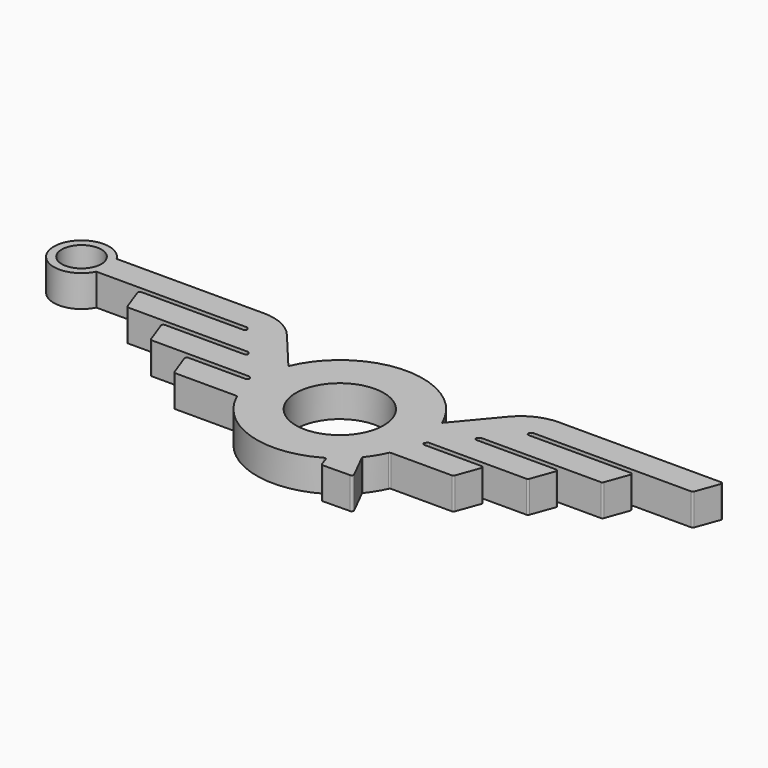
from build123d import *

# Parameters (mm, degrees)
F0_R     = 11.1
F1_DEPTH = 4
F2_DEPTH = 4
F3_DEPTH = 4
F4_DEPTH = 4
F5_R     = 0.5
F6_R     = 7
F6_R_2   = 5
F7_DEPTH = 4
F8_R     = 5
F9_DEPTH = 25
F10_R    = 12


# Not quite as in the source:
# - a feature names something its author has since deleted; it is built from what else it names


with BuildPart() as f1:
    # F0 (on Top) → F1 (new body, symmetric)
    with BuildSketch(Plane.XY):
        with BuildLine():
            ThreePointArc((20.944924, -1.519927), (20.986226, -0.760462), (21, 0))
            ThreePointArc((21, 0), (20.598026, 4.089169), (19.407495, 8.021792))
            ThreePointArc((19.407495, 8.021792), (0, 21), (-19.407495, 8.021792))
            ThreePointArc((-19.407495, 8.021792), (-20.732595, 3.340581), (-20.944924, -1.519927))
            ThreePointArc((-20.944924, -1.519927), (-20.403011, -4.971634), (-19.296293, -8.285714))
            ThreePointArc((-19.296293, -8.285714), (-6.345132, -20.018474), (11, -17.888544))
            ThreePointArc((11, -17.888544), (13.82448, -15.807712), (16.263142, -13.285714))
            ThreePointArc((16.263142, -13.285714), (17.95462, -10.891815), (19.296293, -8.285714))
            ThreePointArc((19.296293, -8.285714), (20.403011, -4.971634), (20.944924, -1.519927))
        make_face()
        Circle(F0_R, mode=Mode.SUBTRACT)
        with BuildLine():
            Line((20, -20.736863), (16.263142, -13.285714))
            ThreePointArc((16.263142, -13.285714), (13.82448, -15.807712), (11, -17.888544))
            Line((11, -17.888544), (12, -20.842855))
            Line((12, -20.842855), (20, -20.736863))
        make_face()
    extrude(amount=F1_DEPTH, both=True)

    # F0 (on Top) → F2 (join, symmetric)
    with BuildSketch(Plane.XY):
        with BuildLine():
            Line((21.466717, -1.519927), (20.944924, -1.519927))
            ThreePointArc((20.944924, -1.519927), (20.403011, -4.971634), (19.296293, -8.285714))
            Line((19.296293, -8.285714), (35.296293, -8.285714))
            Line((35.296293, -8.285714), (37.758838, -1.519927))
            Line((37.758838, -1.519927), (21.466717, -1.519927))
        make_face()
    extrude(amount=F2_DEPTH, both=True)

    # F0 (on Top) → F3 (join, symmetric)
    with BuildSketch(Plane.XY):
        with BuildLine():
            ThreePointArc((19.407495, 8.021792), (20.598026, 4.089169), (21, 0))
            ThreePointArc((21, 0), (20.986226, -0.760462), (20.944924, -1.519927))
            Line((20.944924, -1.519927), (21.466717, -1.519927))
            Line((21.466717, -1.519927), (22.552058, -0.223202))
            Line((22.552058, -0.223202), (22.998917, -0.223202))
            Line((22.998917, -0.223202), (47.674407, -0.223202))
            Line((47.674407, -0.223202), (50.136952, 6.542585))
            Line((50.136952, 6.542585), (29.636583, 6.542585))
            Line((29.636583, 6.542585), (28.214928, 6.542585))
            Line((28.214928, 6.542585), (29.28627, 7.822585))
            Line((29.28627, 7.822585), (47.431346, 7.822585))
            Line((47.431346, 7.822585), (60.054694, 7.822585))
            Line((60.054694, 7.822585), (62.517239, 14.588372))
            Line((62.517239, 14.588372), (43.96666, 14.588372))
            Line((43.96666, 14.588372), (34.94914, 14.588372))
            Line((34.94914, 14.588372), (36.020482, 15.868372))
            Line((36.020482, 15.868372), (54.509119, 15.868372))
            Line((54.509119, 15.868372), (62.740314, 15.868372))
            Line((62.740314, 15.868372), (76.458602, 15.868372))
            Line((76.458602, 15.868372), (78.921147, 22.634159))
            Line((78.921147, 22.634159), (31.637842, 22.634159))
            Line((31.637842, 22.634159), (19.407495, 8.021792))
        make_face()
    extrude(amount=F3_DEPTH, both=True)

    # F0 (on Top) → F4 (join, symmetric)
    with BuildSketch(Plane.XY):
        with BuildLine():
            ThreePointArc((20.944924, -1.519927), (20.986226, -0.760462), (21, 0))
            ThreePointArc((21, 0), (20.598026, 4.089169), (19.407495, 8.021792))
            ThreePointArc((19.407495, 8.021792), (0, 21), (-19.407495, 8.021792))
            ThreePointArc((-19.407495, 8.021792), (-20.732595, 3.340581), (-20.944924, -1.519927))
            ThreePointArc((-20.944924, -1.519927), (-20.403011, -4.971634), (-19.296293, -8.285714))
            ThreePointArc((-19.296293, -8.285714), (-6.345132, -20.018474), (11, -17.888544))
            ThreePointArc((11, -17.888544), (13.82448, -15.807712), (16.263142, -13.285714))
            ThreePointArc((16.263142, -13.285714), (17.95462, -10.891815), (19.296293, -8.285714))
            ThreePointArc((19.296293, -8.285714), (20.403011, -4.971634), (20.944924, -1.519927))
        make_face()
        Circle(F0_R, mode=Mode.SUBTRACT)
        with BuildLine():
            ThreePointArc((19.407495, 8.021792), (20.598026, 4.089169), (21, 0))
            ThreePointArc((21, 0), (20.986226, -0.760462), (20.944924, -1.519927))
            Line((20.944924, -1.519927), (21.466717, -1.519927))
            Line((21.466717, -1.519927), (22.552058, -0.223202))
            Line((22.552058, -0.223202), (22.998917, -0.223202))
            Line((22.998917, -0.223202), (47.674407, -0.223202))
            Line((47.674407, -0.223202), (50.136952, 6.542585))
            Line((50.136952, 6.542585), (29.636583, 6.542585))
            Line((29.636583, 6.542585), (28.214928, 6.542585))
            Line((28.214928, 6.542585), (29.28627, 7.822585))
            Line((29.28627, 7.822585), (47.431346, 7.822585))
            Line((47.431346, 7.822585), (60.054694, 7.822585))
            Line((60.054694, 7.822585), (62.517239, 14.588372))
            Line((62.517239, 14.588372), (43.96666, 14.588372))
            Line((43.96666, 14.588372), (34.94914, 14.588372))
            Line((34.94914, 14.588372), (36.020482, 15.868372))
            Line((36.020482, 15.868372), (54.509119, 15.868372))
            Line((54.509119, 15.868372), (62.740314, 15.868372))
            Line((62.740314, 15.868372), (76.458602, 15.868372))
            Line((76.458602, 15.868372), (78.921147, 22.634159))
            Line((78.921147, 22.634159), (31.637842, 22.634159))
            Line((31.637842, 22.634159), (19.407495, 8.021792))
        make_face()
        with BuildLine():
            Line((21.466717, -1.519927), (20.944924, -1.519927))
            ThreePointArc((20.944924, -1.519927), (20.403011, -4.971634), (19.296293, -8.285714))
            Line((19.296293, -8.285714), (35.296293, -8.285714))
            Line((35.296293, -8.285714), (37.758838, -1.519927))
            Line((37.758838, -1.519927), (21.466717, -1.519927))
        make_face()
        with BuildLine():
            ThreePointArc((-20.944924, -1.519927), (-20.732595, 3.340581), (-19.407495, 8.021792))
            Line((-19.407495, 8.021792), (-31.637842, 22.634159))
            Line((-31.637842, 22.634159), (-78.921147, 22.634159))
            Line((-78.921147, 22.634159), (-76.458602, 15.868372))
            Line((-76.458602, 15.868372), (-62.740314, 15.868372))
            Line((-62.740314, 15.868372), (-54.509119, 15.868372))
            Line((-54.509119, 15.868372), (-36.020482, 15.868372))
            Line((-36.020482, 15.868372), (-34.94914, 14.588372))
            Line((-34.94914, 14.588372), (-43.96666, 14.588372))
            Line((-43.96666, 14.588372), (-62.517239, 14.588372))
            Line((-62.517239, 14.588372), (-60.054694, 7.822585))
            Line((-60.054694, 7.822585), (-47.431346, 7.822585))
            Line((-47.431346, 7.822585), (-29.28627, 7.822585))
            Line((-29.28627, 7.822585), (-28.214928, 6.542585))
            Line((-28.214928, 6.542585), (-29.636583, 6.542585))
            Line((-29.636583, 6.542585), (-50.136952, 6.542585))
            Line((-50.136952, 6.542585), (-47.674407, -0.223202))
            Line((-47.674407, -0.223202), (-22.552058, -0.223202))
            Line((-22.552058, -0.223202), (-21.466717, -1.519927))
            Line((-21.466717, -1.519927), (-20.944924, -1.519927))
        make_face()
        with BuildLine():
            ThreePointArc((-19.296293, -8.285714), (-20.403011, -4.971634), (-20.944924, -1.519927))
            Line((-20.944924, -1.519927), (-21.466717, -1.519927))
            Line((-21.466717, -1.519927), (-37.758838, -1.519927))
            Line((-37.758838, -1.519927), (-35.296293, -8.285714))
            Line((-35.296293, -8.285714), (-19.296293, -8.285714))
        make_face()
        with BuildLine():
            Line((20, -20.736863), (16.263142, -13.285714))
            ThreePointArc((16.263142, -13.285714), (13.82448, -15.807712), (11, -17.888544))
            Line((11, -17.888544), (12, -20.842855))
            Line((12, -20.842855), (20, -20.736863))
        make_face()
    extrude(amount=F4_DEPTH, both=True)

    # F5
    f5_edges = [f1.edges().sort_by_distance(p)[0] for p in [
        (-36.020482, 15.868372, 0),
        (-29.28627, 7.822585, 0),
        (-22.552058, -0.223202, 0),
        (-19.296293, -8.285714, 0),
        (-21.466717, -1.519927, 0),
        (-28.214928, 6.542585, 0),
        (-34.94914, 14.588372, 0),
        (-78.921147, 22.634159, 0),
        (-76.458602, 15.868372, 0),
        (-62.517239, 14.588372, 0),
        (-60.054694, 7.822585, 0),
        (-50.136952, 6.542585, 0),
        (-37.758838, -1.519927, 0),
        (-35.296293, -8.285714, 0),
        (-47.674407, -0.223202, 0),
        (78.921147, 22.634159, 0),
        (76.458602, 15.868372, 0),
        (62.517239, 14.588372, 0),
        (60.054694, 7.822585, 0),
        (50.136952, 6.542585, 0),
        (37.758838, -1.519927, 0),
        (35.296293, -8.285714, 0),
        (47.674407, -0.223202, 0),
        (21.466717, -1.519927, 0),
        (28.214928, 6.542585, 0),
        (34.94914, 14.588372, 0),
        (36.020482, 15.868372, 0),
        (29.28627, 7.822585, 0),
        (22.552058, -0.223202, 0),
        (19.296293, -8.285714, 0),
        (20, -20.736863, 0),
        (12, -20.842855, 0),
        (11, -17.888544, 0),
        (16.263142, -13.285714, 0),
    ]]
    fillet(f5_edges, radius=F5_R)

    # F6 (on Top) → F7 (join, symmetric)
    with BuildSketch(Plane.XY):
        with Locations((-80.473438, 19.015618)):
            Circle(F6_R)
        with Locations((-80.473438, 19.015618)):
            Circle(F6_R_2, mode=Mode.SUBTRACT)
    extrude(amount=F7_DEPTH, both=True)

    # F8 (on face) → F9 (cut)
    with BuildSketch(Plane.XY.offset(4)):
        with Locations((-80.473438, 19.015618)):
            Circle(F8_R)
    extrude(amount=-F9_DEPTH, mode=Mode.SUBTRACT)

    # F10
    f10_edges = [f1.edges().sort_by_distance(p)[0] for p in [
        (-31.637842, 22.634159, 0),
        (31.637842, 22.634159, 0),
    ]]
    fillet(f10_edges, radius=F10_R)


solid = f1.part
